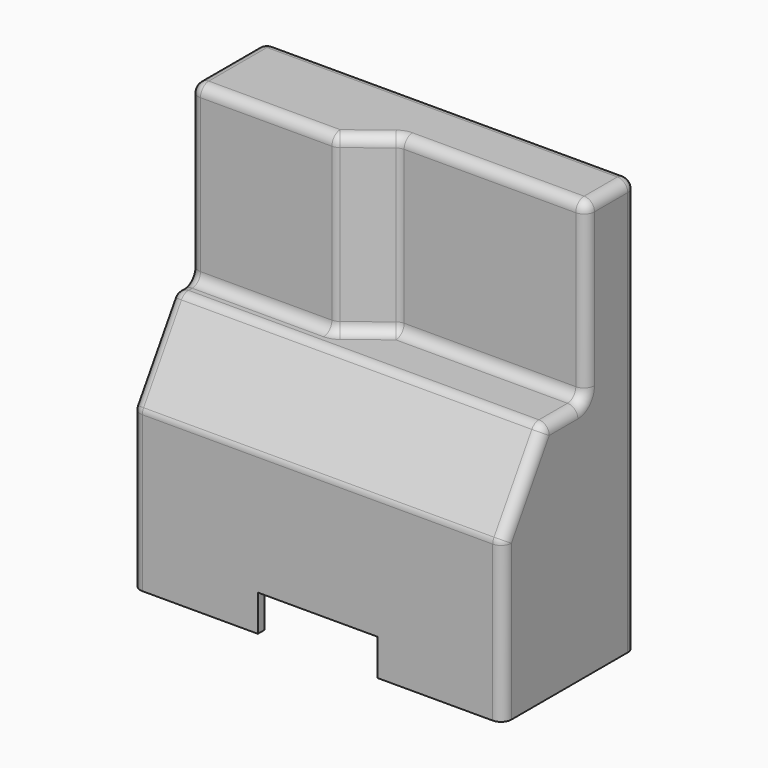
from build123d import *

# Parameters (mm, degrees)
F0_W      = 71.5
F0_H      = 32
F1_DEPTH  = 30.5
F3_DEPTH  = 35.75
F4_W      = 12
F4_H      = 33.5
F5_DEPTH  = 35.75
F7_DEPTH  = 80
F8_R      = 2
F9_T      = -1.6
F10_W     = 23
F10_H     = 14
F11_DEPTH = 25


with BuildPart() as f1:
    # F0 (on Top) → F1 (new body)
    with BuildSketch(Plane.XY):
        Rectangle(F0_W, F0_H)
    extrude(amount=F1_DEPTH)

    # F2 (on Right) → F3 (join, symmetric)
    with BuildSketch(Plane.YZ):
        Polygon((-16, 30.5), (0, 30.5), (16, 30.5), (16, 46.5), (-6, 46.5), align=None)
    extrude(amount=F3_DEPTH, both=True)

    # F4 (on Right) → F5 (join, symmetric)
    with BuildSketch(Plane.YZ):
        with Locations((10, 63.25)):
            Rectangle(F4_W, F4_H)
    extrude(amount=F5_DEPTH, both=True)

    # F6 (on Top) → F7 (join)
    with BuildSketch(Plane.XY):
        Polygon((-7.75, -2), (0, 4), (0, 16), (-35.75, 16), (-35.75, -2), align=None)
    extrude(amount=F7_DEPTH)

    # F8
    f8_edges = [f1.edges().sort_by_distance(p)[0] for p in [
        (0, 4, 63.25),
        (-7.75, -2, 63.25),
        (17.875, 4, 46.5),
        (0, -6, 46.5),
        (0, -16, 30.5),
        (35.75, 4, 63.25),
        (35.75, 16, 40),
        (0, 16, 80),
        (35.75, 10, 80),
        (17.875, 4, 80),
        (-21.75, -2, 80),
        (-35.75, 7, 80),
        (-35.75, -2, 63.25),
        (-35.75, 16, 40),
        (-35.75, -11, 38.5),
        (-35.75, -16, 15.25),
        (-35.75, -4, 46.5),
        (35.75, -11, 38.5),
        (35.75, -16, 15.25),
        (-21.75, -2, 46.5),
        (35.75, -1, 46.5),
        (-3.875, 1, 46.5),
        (-3.875, 1, 80),
    ]]
    fillet(f8_edges, radius=F8_R)

    # F9
    f9_openings = [f1.faces().sort_by_distance(p)[0] for p in [
        (0, 0, 0),
    ]]
    offset(amount=F9_T, openings=f9_openings)


with BuildPart() as f11:
    # F10 (on Front) → F11 (new body)
    with BuildSketch(Plane.XZ):
        Rectangle(F10_W, F10_H)
    extrude(amount=F11_DEPTH)


with BuildPart() as f1_1:
    add(f1.part)

    # F12: cut F11
    add(f11.part, mode=Mode.SUBTRACT)


solid = f1_1.part
